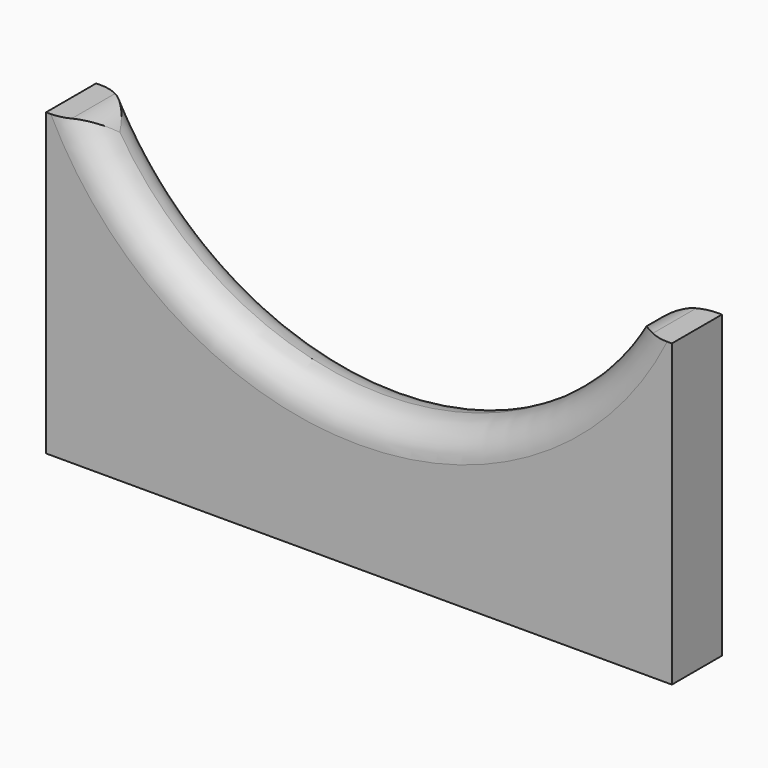
from build123d import *

# Parameters (mm, degrees)
F1_DEPTH = 25
F2_R     = 12.49999


# Not quite as in the source:
# - a fillet or chamfer is up to 0.001 mm smaller than in the source, because OpenCascade refuses the exact size


with BuildPart() as f1:
    # F0 (on Front) → F1 (new body)
    with BuildSketch(Plane.XZ):
        with BuildLine():
            Line((-277.959928672, -3.7163552741), (-277.959928672, -123.7163552741))
            Line((-277.959928672, -123.7163552741), (-27.959928672, -123.7163552741))
            Line((-27.959928672, -123.7163552741), (-27.959928672, -3.7163552741))
            Line((-27.959928672, -3.7163552741), (-43.9558270226, -3.7163552741))
            ThreePointArc((-43.9558270226, -3.7163552741), (-152.9567080066, -67.529690512), (-261.9575889906, -3.7163552741))
            Line((-261.9575889906, -3.7163552741), (-277.959928672, -3.7163552741))
        make_face()
    extrude(amount=F1_DEPTH)

    # F2 (radius 12.5 in the source; OpenCascade refuses exactly that, so slightly less here)
    f2_edges = [f1.edges().sort_by_distance(p)[0] for p in [
        (-261.957589, -12.5, -3.716355),
        (-43.955827, -12.5, -3.716355),
        (-152.956708, -25, -67.529691),
        (-152.956708, 0, -67.529691),
    ]]
    fillet(f2_edges, radius=F2_R)


solid = f1.part
